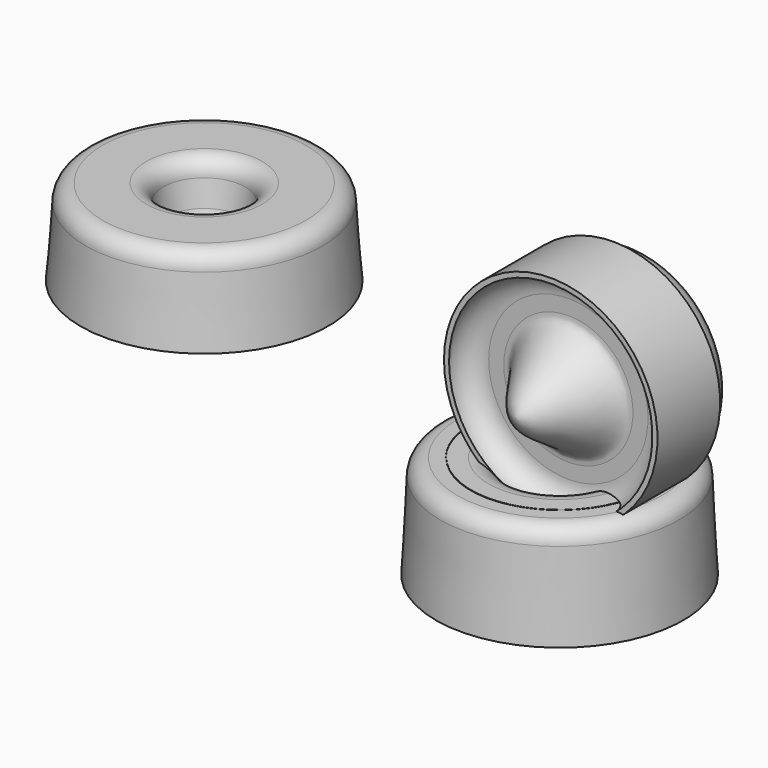
from build123d import *

# Parameters (mm, degrees)
F6_R     = 25
F7_R     = 52.5
F7_R_2   = 52.2
F8_DEPTH = 0.3


with BuildPart() as f1:
    # F0 (on Top) → F1 (revolve)
    with BuildSketch(Plane.XY):
        with BuildLine():
            Line((-19.05, 0), (-19.05, 19.05))
            ThreePointArc((-19.05, 19.05), (-24.6296158184, 32.5203841816), (-38.1, 38.1))
            Line((-38.1, 38.1), (-40.95, 38.1))
            ThreePointArc((-40.95, 38.1), (-54.4203841816, 32.5203841816), (-60, 19.05))
            Line((-60, 19.05), (-60, 20.5188412219))
            Line((-60, 20.5188412219), (-63, 20.5188412219))
            Line((-63, 20.5188412219), (-63, -25.7))
            Line((-63, -25.7), (-60, -25.7))
            ThreePointArc((-60, -25.7), (-56.1923881554, -16.5076118446), (-47, -12.7))
            Line((-47, -12.7), (-38.1042405314, -12.7))
            add(Edge.make_bspline(
                [(0, -50.8), (-2.0822347318, -50.9101227966), (-7.1940842075, -48.1763778773), (-12.5245183089, -43.2045045711), (-17.9918415298, -35.4682218921), (-25.3032798984, -24.8614897261), (-32.8278460834, -13.4604600665), (-36.1188747437, -12.7), (-38.1042405314, -12.7)],
                knots=[0, 0, 0, 0, 0.1500756453, 0.301860001, 0.4706002275, 0.6765659, 0.8766479175, 1, 1, 1, 1], degree=3))
            Line((0, -50.8), (0, -19.05))
            ThreePointArc((0, -19.05), (-13.4703841816, -13.4703841816), (-19.05, 0))
        make_face()
    revolve(axis=Axis((0, -4.1539501399, 0), (0, -1, 0)))


with BuildPart() as f3:
    # F2 (on Front) → F3 (revolve)
    with BuildSketch(Plane.XZ):
        with BuildLine():
            ThreePointArc((-249.2126121662, 18.7093689321), (-252.1415443543, 25.780436744), (-259.2126121662, 28.7093689321))
            Line((-259.2126121662, 28.7093689321), (-285.0126121662, 28.7093689321))
            ThreePointArc((-285.0126121662, 28.7093689321), (-292.0836799781, 25.780436744), (-295.0126121662, 18.7093689321))
            Line((-295.0126121662, 18.7093689321), (-298.0126121662, -22.0906310679))
            Line((-298.0126121662, -22.0906310679), (-295.0126121662, -22.0906310679))
            ThreePointArc((-295.0126121662, -22.0906310679), (-292.0836799781, -15.019563256), (-285.0126121662, -12.0906310679))
            Line((-285.0126121662, -12.0906310679), (-259.2126121662, -12.0906310679))
            ThreePointArc((-259.2126121662, -12.0906310679), (-252.1415443543, -15.019563256), (-249.2126121662, -22.0906310679))
            add(Edge.make_bspline(
                [(-247.2126121662, -36.9646690271), (-247.6035198675, -34.1473602606), (-248.2930925928, -29.0470066466), (-248.9341250638, -24.8754665916), (-249.2126121662, -22.0906310679)],
                knots=[0, 0, 0, 0, 0.5123688981, 1, 1, 1, 1], degree=3))
            ThreePointArc((-247.2126121662, -36.9646690271), (-245.7253366676, -40.9549919208), (-242.7126121662, -43.9646690271))
            ThreePointArc((-242.7126121662, -43.9646690271), (-233.9888307464, -46.2093586504), (-225.0126121662, -46.9646690271))
            Line((-225.0126121662, -46.9646690271), (-225.0126121662, -6.1646690271))
            ThreePointArc((-225.0126121662, -6.1646690271), (-233.9888307464, -5.4093586504), (-242.7126121662, -3.1646690271))
            ThreePointArc((-242.7126121662, -3.1646690271), (-245.7253366676, -0.1549919208), (-247.2126121662, 3.8353309729))
            add(Edge.make_bspline(
                [(-249.2126121662, 18.7093689321), (-248.948773219, 16.3656932526), (-248.1100526093, 11.6257684469), (-247.6175158399, 6.4486636586), (-247.2126121662, 3.8353309729)],
                knots=[0, 0, 0, 0, 0.4880084671, 1, 1, 1, 1], degree=3))
        make_face()
    revolve(axis=Axis((-225.0126121662, 0, -26.5646690271), (0, 0, -1)))


with BuildPart() as f5:
    # F4 (on Front) → F5 (revolve)
    with BuildSketch(Plane.XZ):
        with BuildLine():
            Line((-15.3189936567, -131.602422893), (-15.3189936567, -80.802422893))
            ThreePointArc((-15.3189936567, -80.802422893), (-24.4093316446, -80.0732931242), (-33.2453176379, -77.8169184923))
            ThreePointArc((-33.2453176379, -77.8169184923), (-36.9105601831, -75.3213480939), (-39.1364358366, -71.4863315225))
            add(Edge.make_bspline(
                [(-42.3189936567, -60.802422893), (-41.710263485, -62.7006069208), (-41.1481836805, -66.8323165607), (-39.9121455848, -69.6763470769), (-39.1364358366, -71.4863315225)],
                knots=[0, 0, 0, 0, 0.5183761675, 1, 1, 1, 1], degree=3))
            ThreePointArc((-42.3189936567, -60.802422893), (-46.7123919389, -50.1958211752), (-57.3189936567, -45.802422893))
            Line((-57.3189936567, -45.802422893), (-75.8002488929, -45.802422893))
            ThreePointArc((-75.8002488929, -45.802422893), (-82.6948766947, -48.5592117629), (-85.7880978592, -55.309601398))
            Line((-85.7880978592, -55.309601398), (-88.3189936567, -106.602422893))
            Line((-88.3189936567, -106.602422893), (-85.3189936567, -106.602422893))
            Line((-85.3189936567, -106.602422893), (-82.3189936567, -106.602422893))
            ThreePointArc((-82.3189936567, -106.602422893), (-79.3900614686, -99.5313550812), (-72.3189936567, -96.602422893))
            Line((-72.3189936567, -96.602422893), (-49.5189936567, -96.602422893))
            ThreePointArc((-49.5189936567, -96.602422893), (-42.4479258448, -99.5313550812), (-39.5189936567, -106.602422893))
            add(Edge.make_bspline(
                [(-37.6314280629, -121.6553889513), (-38.0201655406, -118.8537211917), (-38.7797640016, -113.7620469567), (-39.2388820282, -109.4035034713), (-39.5189936567, -106.602422893)],
                knots=[0, 0, 0, 0, 0.5095243517, 1, 1, 1, 1], degree=3))
            ThreePointArc((-37.6314280629, -121.6553889513), (-36.1441525644, -125.6457118451), (-33.1314280629, -128.6553889513))
            ThreePointArc((-33.1314280629, -128.6553889513), (-24.3499166083, -130.8826512166), (-15.3189936567, -131.602422893))
        make_face()
    revolve(axis=Axis((-15.3189936567, 0, -106.202422893), (0, 0, -1)))

    # F6
    f6_edges = [f5.edges().sort_by_distance(p)[0] for p in [
        (11.681006, 0, -60.802423),
        (8.498449, 0, -71.486332),
    ]]
    fillet(f6_edges, radius=F6_R)

    # F7 (on face) → F8 (cut)
    with BuildSketch(Plane.XY.offset(-45.802422893)):
        with Locations((-15.3189936567, 0)):
            Circle(F7_R)
        with Locations((-15.3189936567, 0)):
            Circle(F7_R_2, mode=Mode.SUBTRACT)
    extrude(amount=-F8_DEPTH, mode=Mode.SUBTRACT)


solid = Compound([f1.part, f3.part, f5.part])
